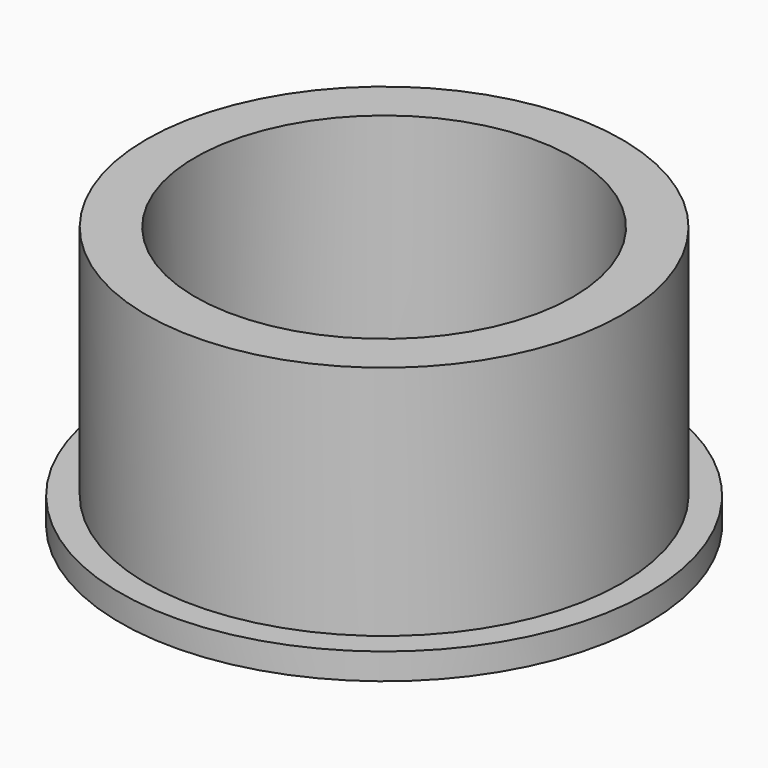
from build123d import *

# Parameters (mm, degrees)
F1_R     = 31.9405
F1_R_2   = 28.7655
F2_DEPTH = 3.175
F1_R_3   = 22.86
F3_DEPTH = 31.75


# Not quite as in the source:
# - a variable given as a bare number and used for a length is read in inches; the dataset says mm whatever the document's units were


with BuildPart() as f2:
    # F1 (on Top) → F2 (new body)
    with BuildSketch(Plane.XY):
        Circle(F1_R)
        Circle(F1_R_2, mode=Mode.SUBTRACT)
    extrude(amount=F2_DEPTH)

    # F1 (on Top) → F3 (join)
    with BuildSketch(Plane.XY):
        Circle(F1_R_2)
        Circle(F1_R_3, mode=Mode.SUBTRACT)
    extrude(amount=F3_DEPTH)


solid = f2.part
